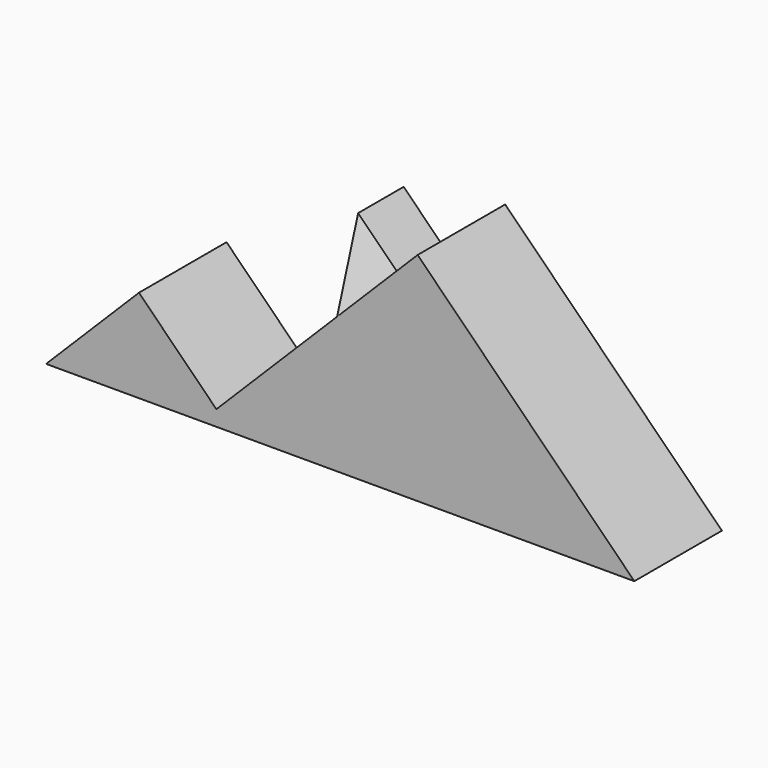
from build123d import *

# Parameters (mm, degrees)
F1_DEPTH    = 25
F2_T1_DEPTH = 46.6847527524
F3_SIZE     = 12.99999


# Not quite as in the source:
# - a fillet or chamfer that OpenCascade refuses, or shapes differently, is made with other operations: its cross-section is extruded or revolved along the edge and cut away or added
# - a fillet or chamfer is up to 0.001 mm smaller than in the source, because OpenCascade refuses the exact size


with BuildPart() as f1:
    # F0 (on Front) → F1 (new body)
    with BuildSketch(Plane.XZ):
        Polygon((21.2132034356, 21.2132034356), (0, 0), (134.3502884254, 0), (84.8528137424, 49.4974746831), (75.660425587, 40.3050865276), (66.4680374315, 31.1126983722), (56.5685424949, 21.2132034356), (38.8908729653, 3.5355339059), align=None)
        Polygon((66.4680374315, 31.1126983722), (75.660425587, 40.3050865276), (66.4680374315, 49.4974746831), (57.2756492761, 40.3050865276), align=None)
    extrude(amount=F1_DEPTH)

    # F2: chamfer of 6 x 13 on 2 edges, made by hand

    # F2_s2 → F2_t1 (cut)
    with BuildSketch(Plane(origin=(17.6776695297, 0, -17.6776695297), x_dir=(0, 1, 0), z_dir=(-0.7071067812, 0, 0.7071067812))):
        Polygon((-19, -82), (-25, -69), (-25, -82), align=None)
        Polygon((-6, -82), (0, -69), (0, -82), align=None)
    extrude(amount=F2_T1_DEPTH, mode=Mode.SUBTRACT)

    # F3 (size 13 in the source; OpenCascade refuses exactly that, so slightly less here)
    f3_edges = [f1.edges().sort_by_distance(p)[0] for p in [
        (57.275649, -12.5, 40.305087),
    ]]
    chamfer(f3_edges, length=F3_SIZE)


solid = f1.part
